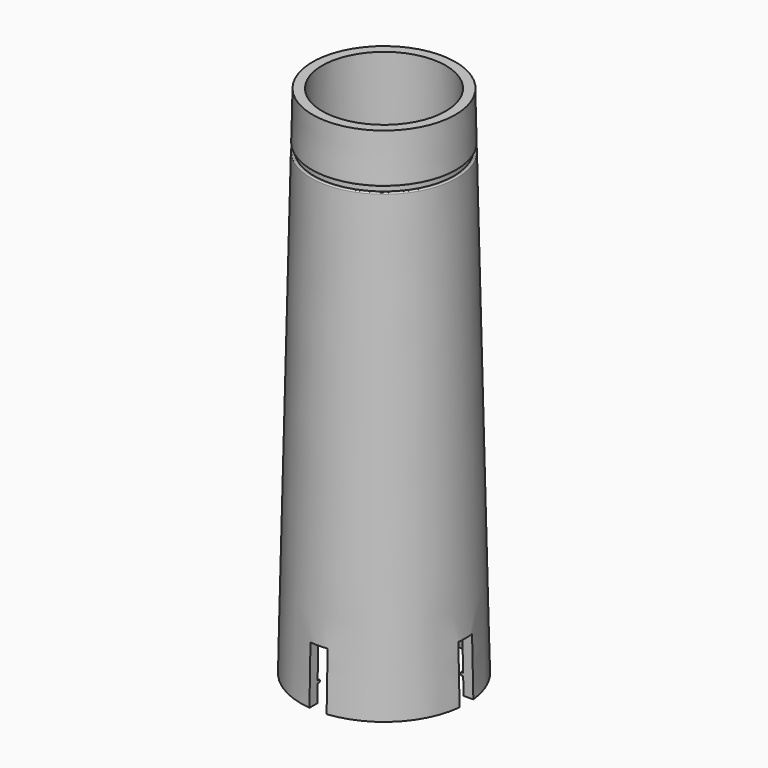
from build123d import *

# Parameters (mm, degrees)
F0_R          = 14.5
F2_R          = 12.5
F5_R          = 10.8
F4_R          = 12.8
F8_R          = 14.5
F8_R_2        = 12.25
F9_DEPTH      = 0.5
F10_DEPTH     = 0.5
F11_R         = 0.2
F13_R         = 14
F13_R_2       = 12.2
F14_DEPTH     = 0.5
F15_DEPTH     = 0.5
F16_W         = 3
F16_H         = 15
F16_H_2       = 3
F16_W_2       = 15
F17_DEPTH     = 10
F18_T2_ANGLE  = 82.921707092
F18_T4_ANGLE  = 82.921707092
F18_T6_ANGLE  = 82.921707092
F18_T8_ANGLE  = 82.921707092
F18_T10_ANGLE = 82.921707092
F18_T12_ANGLE = 82.921707092
F18_T14_ANGLE = 82.921707092
F18_T16_ANGLE = 82.921707092


# Not quite as in the source:
# - a fillet or chamfer that OpenCascade refuses, or shapes differently, is made with other operations: its cross-section is extruded or revolved along the edge and cut away or added
# - a feature of the source that left no trace in its solid (it failed there, or was rolled back) is left out


with BuildPart() as f3:
    # F0 (on Top) → F3 section 0
    with BuildSketch(Plane.XY):
        Circle(F0_R)
    # F2 (on offset) → F3 section 1
    with BuildSketch(Plane.XY.offset(90)):
        Circle(F2_R)
    loft()

    # F5 (on face) → F6 section 0
    with BuildSketch(Plane.XY.offset(90)):
        Circle(F5_R)
    # F4 (on Top) → F6 section 1
    with BuildSketch(Plane.XY):
        Circle(F4_R)
    loft(mode=Mode.SUBTRACT)

    # F8 (on offset) → F9 (cut)
    with BuildSketch(Plane.XY.offset(81)):
        Circle(F8_R)
        Circle(F8_R_2, mode=Mode.SUBTRACT)
    extrude(amount=F9_DEPTH, mode=Mode.SUBTRACT)

    # F8 (on offset) → F10 (cut)
    with BuildSketch(Plane.XY.offset(81)):
        Circle(F8_R)
        Circle(F8_R_2, mode=Mode.SUBTRACT)
    extrude(amount=-F10_DEPTH, mode=Mode.SUBTRACT)

    # F11
    f11_edges = [f3.edges().sort_by_distance(p)[0] for p in [
        (-12.711111, 0, 80.5),
        (-12.688889, 0, 81.5),
    ]]
    fillet(f11_edges, radius=F11_R)

    # F13 (on offset) → F14 (join)
    with BuildSketch(Plane.XY.offset(3)):
        Circle(F13_R)
        Circle(F13_R_2, mode=Mode.SUBTRACT)
    extrude(amount=F14_DEPTH)

    # F13 (on offset) → F15 (join)
    with BuildSketch(Plane.XY.offset(3)):
        Circle(F13_R)
        Circle(F13_R_2, mode=Mode.SUBTRACT)
    extrude(amount=F15_DEPTH)

    # F16 (on face) → F17 (cut)
    with BuildSketch(Plane.XY):
        with Locations((0, 9)):
            Rectangle(F16_W, F16_H)
        Rectangle(F16_W, F16_H_2)
        with Locations((-9, 0)):
            Rectangle(F16_W_2, F16_H_2)
        with Locations((9, 0)):
            Rectangle(F16_W_2, F16_H_2)
        with Locations((0, -9)):
            Rectangle(F16_W, F16_H)
    extrude(amount=F17_DEPTH, mode=Mode.SUBTRACT)

    # F18: fillet of radius 0.3 on 8 edges, made by hand

    # F18_s1 → F18_t2 (revolve, cut)
    with BuildSketch(Plane(origin=(0, 0, 0), x_dir=(0, 0, 1), z_dir=(-0.0617304854, 0.998092855, 0))):
        with BuildLine():
            ThreePointArc((3.3, -12.2), (3.0878679656, -12.2878679656), (3, -12.5))
            Line((3, -12.5), (3, -12.2))
            Line((3, -12.2), (3.3, -12.2))
        make_face()
    revolve(axis=Axis((0, 0, 3), (0, 0, 1)), revolution_arc=F18_T2_ANGLE, mode=Mode.SUBTRACT)

    # F18_s3 → F18_t4 (revolve, cut)
    with BuildSketch(Plane(origin=(0, 0, 0), x_dir=(0, 0, 1), z_dir=(-0.0617304854, 0.998092855, 0))):
        with BuildLine():
            ThreePointArc((3.5, -12.5), (3.4121320344, -12.2878679656), (3.2, -12.2))
            Line((3.2, -12.2), (3.5, -12.2))
            Line((3.5, -12.2), (3.5, -12.5))
        make_face()
    revolve(axis=Axis((0, 0, 3.5), (0, 0, 1)), revolution_arc=F18_T4_ANGLE, mode=Mode.SUBTRACT)

    # F18_s5 → F18_t6 (revolve, cut)
    with BuildSketch(Plane(origin=(0, 0, 0), x_dir=(0, 0, 1), z_dir=(-0.998092855, -0.0617304854, 0))):
        with BuildLine():
            ThreePointArc((3.3, -12.2), (3.0878679656, -12.2878679656), (3, -12.5))
            Line((3, -12.5), (3, -12.2))
            Line((3, -12.2), (3.3, -12.2))
        make_face()
    revolve(axis=Axis((0, 0, 3), (0, 0, 1)), revolution_arc=F18_T6_ANGLE, mode=Mode.SUBTRACT)

    # F18_s7 → F18_t8 (revolve, cut)
    with BuildSketch(Plane(origin=(0, 0, 0), x_dir=(0, 0, 1), z_dir=(-0.998092855, -0.0617304854, 0))):
        with BuildLine():
            ThreePointArc((3.5, -12.5), (3.4121320344, -12.2878679656), (3.2, -12.2))
            Line((3.2, -12.2), (3.5, -12.2))
            Line((3.5, -12.2), (3.5, -12.5))
        make_face()
    revolve(axis=Axis((0, 0, 3.5), (0, 0, 1)), revolution_arc=F18_T8_ANGLE, mode=Mode.SUBTRACT)

    # F18_s9 → F18_t10 (revolve, cut)
    with BuildSketch(Plane(origin=(0, 0, 0), x_dir=(0, 0, 1), z_dir=(0.0617304854, -0.998092855, 0))):
        with BuildLine():
            ThreePointArc((3.3, -12.2), (3.0878679656, -12.2878679656), (3, -12.5))
            Line((3, -12.5), (3, -12.2))
            Line((3, -12.2), (3.3, -12.2))
        make_face()
    revolve(axis=Axis((0, 0, 3), (0, 0, 1)), revolution_arc=F18_T10_ANGLE, mode=Mode.SUBTRACT)

    # F18_s11 → F18_t12 (revolve, cut)
    with BuildSketch(Plane(origin=(0, 0, 0), x_dir=(0, 0, 1), z_dir=(0.0617304854, -0.998092855, 0))):
        with BuildLine():
            ThreePointArc((3.5, -12.5), (3.4121320344, -12.2878679656), (3.2, -12.2))
            Line((3.2, -12.2), (3.5, -12.2))
            Line((3.5, -12.2), (3.5, -12.5))
        make_face()
    revolve(axis=Axis((0, 0, 3.5), (0, 0, 1)), revolution_arc=F18_T12_ANGLE, mode=Mode.SUBTRACT)

    # F18_s13 → F18_t14 (revolve, cut)
    with BuildSketch(Plane(origin=(0, 0, 0), x_dir=(0, 0, 1), z_dir=(0.998092855, 0.0617304854, 0))):
        with BuildLine():
            ThreePointArc((3.3, -12.2), (3.0878679656, -12.2878679656), (3, -12.5))
            Line((3, -12.5), (3, -12.2))
            Line((3, -12.2), (3.3, -12.2))
        make_face()
    revolve(axis=Axis((0, 0, 3), (0, 0, 1)), revolution_arc=F18_T14_ANGLE, mode=Mode.SUBTRACT)

    # F18_s15 → F18_t16 (revolve, cut)
    with BuildSketch(Plane(origin=(0, 0, 0), x_dir=(0, 0, 1), z_dir=(0.998092855, 0.0617304854, 0))):
        with BuildLine():
            ThreePointArc((3.5, -12.5), (3.4121320344, -12.2878679656), (3.2, -12.2))
            Line((3.2, -12.2), (3.5, -12.2))
            Line((3.5, -12.2), (3.5, -12.5))
        make_face()
    revolve(axis=Axis((0, 0, 3.5), (0, 0, 1)), revolution_arc=F18_T16_ANGLE, mode=Mode.SUBTRACT)


solid = f3.part
